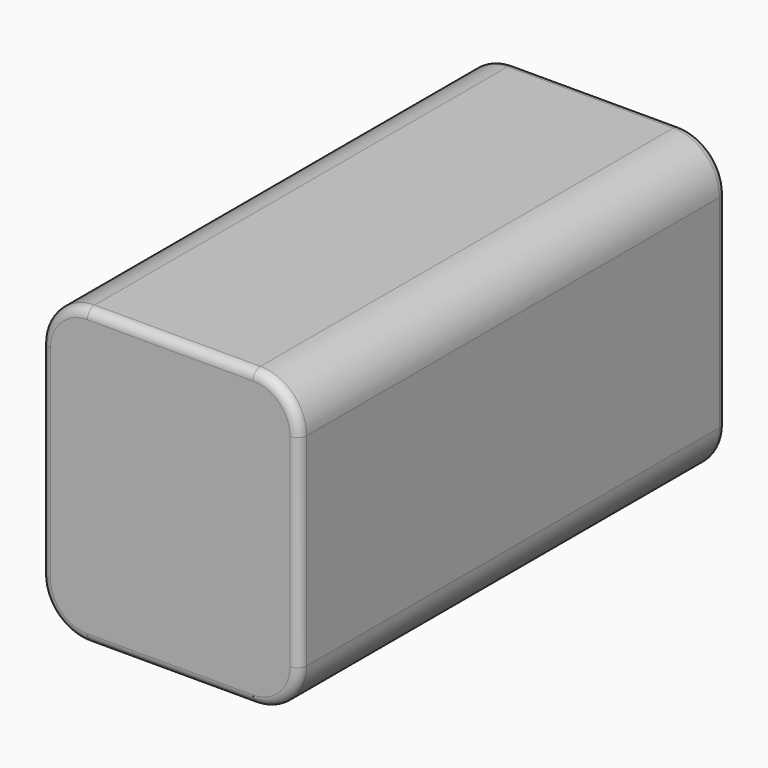
from build123d import *

# Parameters (mm, degrees)
F0_W         = 28
F0_H         = 32
F1_DEPTH     = 58
F2_R         = 1
F3_T1_DEPTH  = 58
F3_T4_ANGLE  = 90
F3_T6_ANGLE  = 90
F3_T8_ANGLE  = 90
F3_T10_ANGLE = 90
F3_T12_ANGLE = 90
F3_T14_ANGLE = 90
F3_T16_ANGLE = 90
F3_T18_ANGLE = 90


# Not quite as in the source:
# - a fillet or chamfer that OpenCascade refuses, or shapes differently, is made with other operations: its cross-section is extruded or revolved along the edge and cut away or added


with BuildPart() as f1:
    # F0 (on Front) → F1 (new body)
    with BuildSketch(Plane.XZ):
        Rectangle(F0_W, F0_H)
    extrude(amount=F1_DEPTH)

    # F2
    f2_edges = [f1.edges().sort_by_distance(p)[0] for p in [
        (0, -58, 16),
        (14, -58, 0),
        (0, -58, -16),
        (-14, -58, 0),
        (14, 0, 0),
        (0, 0, 16),
        (0, 0, -16),
        (-14, 0, 0),
    ]]
    fillet(f2_edges, radius=F2_R)

    # F3: fillet of radius 5 on 4 edges, made by hand

    # F3_s2 → F3_t1 (cut)
    with BuildSketch(Plane.XZ):
        with BuildLine():
            ThreePointArc((9, 16), (12.5355339059, 14.5355339059), (14, 11))
            Line((14, 11), (14, 16))
            Line((14, 16), (9, 16))
        make_face()
        with BuildLine():
            ThreePointArc((-9, 16), (-12.5355339059, 14.5355339059), (-14, 11))
            Line((-14, 11), (-14, 16))
            Line((-14, 16), (-9, 16))
        make_face()
        with BuildLine():
            ThreePointArc((14, -11), (12.5355339059, -14.5355339059), (9, -16))
            Line((9, -16), (14, -16))
            Line((14, -16), (14, -11))
        make_face()
        with BuildLine():
            ThreePointArc((-14, -11), (-12.5355339059, -14.5355339059), (-9, -16))
            Line((-9, -16), (-14, -16))
            Line((-14, -16), (-14, -11))
        make_face()
    extrude(amount=F3_T1_DEPTH, mode=Mode.SUBTRACT)

    # F3_s3 → F3_t4 (revolve, cut)
    with BuildSketch(Plane.YZ.offset(-9)):
        with BuildLine():
            ThreePointArc((0, -15), (-0.2928932188, -15.7071067812), (-1, -16))
            Line((-1, -16), (0, -16))
            Line((0, -16), (0, -15))
        make_face()
    revolve(axis=Axis((-9, 0, -11), (0, 1, 0)), revolution_arc=F3_T4_ANGLE, mode=Mode.SUBTRACT)

    # F3_s5 → F3_t6 (revolve, cut)
    with BuildSketch(Plane.XY.offset(-11)):
        with BuildLine():
            ThreePointArc((-13, -58), (-13.7071067812, -57.7071067812), (-14, -57))
            Line((-14, -57), (-14, -58))
            Line((-14, -58), (-13, -58))
        make_face()
    revolve(axis=Axis((-9, -58, -11), (0, -1, 0)), revolution_arc=F3_T6_ANGLE, mode=Mode.SUBTRACT)

    # F3_s7 → F3_t8 (revolve, cut)
    with BuildSketch(Plane.XY.offset(-11)):
        with BuildLine():
            ThreePointArc((13, 0), (13.7071067812, -0.2928932188), (14, -1))
            Line((14, -1), (14, 0))
            Line((14, 0), (13, 0))
        make_face()
    revolve(axis=Axis((9, 0, -11), (0, 1, 0)), revolution_arc=F3_T8_ANGLE, mode=Mode.SUBTRACT)

    # F3_s9 → F3_t10 (revolve, cut)
    with BuildSketch(Plane.YZ.offset(9)):
        with BuildLine():
            ThreePointArc((-58, -15), (-57.7071067812, -15.7071067812), (-57, -16))
            Line((-57, -16), (-58, -16))
            Line((-58, -16), (-58, -15))
        make_face()
    revolve(axis=Axis((9, -58, -11), (0, -1, 0)), revolution_arc=F3_T10_ANGLE, mode=Mode.SUBTRACT)

    # F3_s11 → F3_t12 (revolve, cut)
    with BuildSketch(Plane.XY.offset(11)):
        with BuildLine():
            ThreePointArc((-13, 0), (-13.7071067812, -0.2928932188), (-14, -1))
            Line((-14, -1), (-14, 0))
            Line((-14, 0), (-13, 0))
        make_face()
    revolve(axis=Axis((-9, 0, 11), (0, 1, 0)), revolution_arc=F3_T12_ANGLE, mode=Mode.SUBTRACT)

    # F3_s13 → F3_t14 (revolve, cut)
    with BuildSketch(Plane.YZ.offset(-9)):
        with BuildLine():
            ThreePointArc((-58, 15), (-57.7071067812, 15.7071067812), (-57, 16))
            Line((-57, 16), (-58, 16))
            Line((-58, 16), (-58, 15))
        make_face()
    revolve(axis=Axis((-9, -58, 11), (0, -1, 0)), revolution_arc=F3_T14_ANGLE, mode=Mode.SUBTRACT)

    # F3_s15 → F3_t16 (revolve, cut)
    with BuildSketch(Plane.YZ.offset(9)):
        with BuildLine():
            ThreePointArc((0, 15), (-0.2928932188, 15.7071067812), (-1, 16))
            Line((-1, 16), (0, 16))
            Line((0, 16), (0, 15))
        make_face()
    revolve(axis=Axis((9, 0, 11), (0, 1, 0)), revolution_arc=F3_T16_ANGLE, mode=Mode.SUBTRACT)

    # F3_s17 → F3_t18 (revolve, cut)
    with BuildSketch(Plane.XY.offset(11)):
        with BuildLine():
            ThreePointArc((13, -58), (13.7071067812, -57.7071067812), (14, -57))
            Line((14, -57), (14, -58))
            Line((14, -58), (13, -58))
        make_face()
    revolve(axis=Axis((9, -58, 11), (0, -1, 0)), revolution_arc=F3_T18_ANGLE, mode=Mode.SUBTRACT)


solid = f1.part
